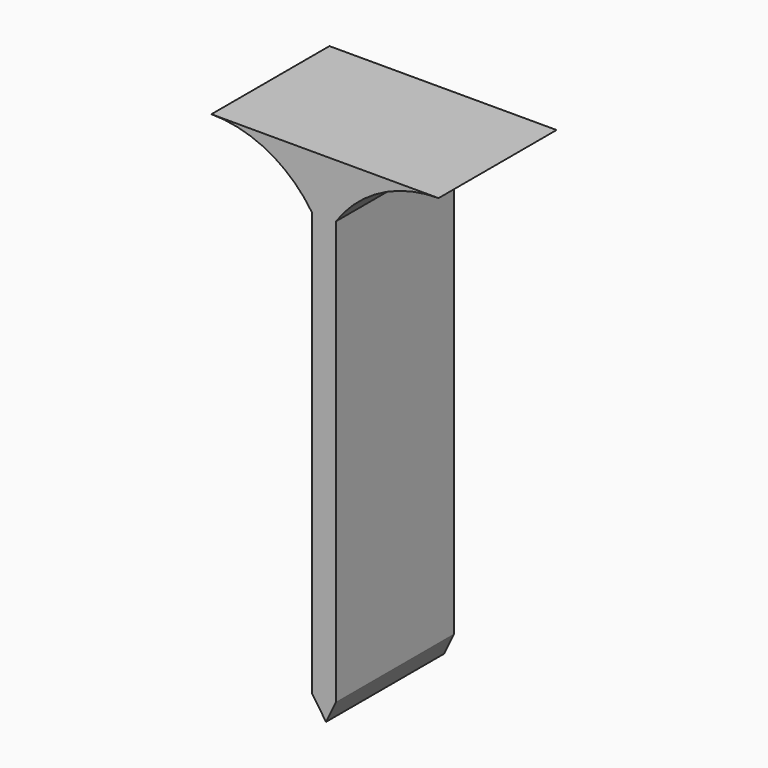
from build123d import *

# Parameters (mm, degrees)
F1_DEPTH = 25.4


# Not quite as in the source:
# - ends of sketch curves that miss each other by under 0.0002 mm in the source are joined


with BuildPart() as f1:
    # F0 (on Front) → F1 (new body)
    with BuildSketch(Plane.XZ):
        Polygon((-2.4299337529, 26.016831398), (-2.4299337529, -46.8811690807), (1.718732994, -46.8811690807), (1.718732994, 26.0008927435), (1.7185925992, 26.0008932828), align=None)
        Polygon((1.718732994, -46.8811690807), (-2.4299337529, -46.8811690807), (0, -50.4371710122), align=None)
        with BuildLine():
            ThreePointArc((-19.7358001024, 35.2624356747), (-9.9254202862, 32.8061351822), (-2.4299337529, 26.016831398))
            Line((-2.4299337529, 26.016831398), (1.7185925992, 26.0008932828))
            ThreePointArc((1.7185925992, 26.0008932828), (9.4088856226, 32.8066016945), (19.3802025169, 35.2624356747))
            Line((19.3802025169, 35.2624356747), (-19.7358001024, 35.2624356747))
        make_face()
    extrude(amount=F1_DEPTH)


solid = f1.part
